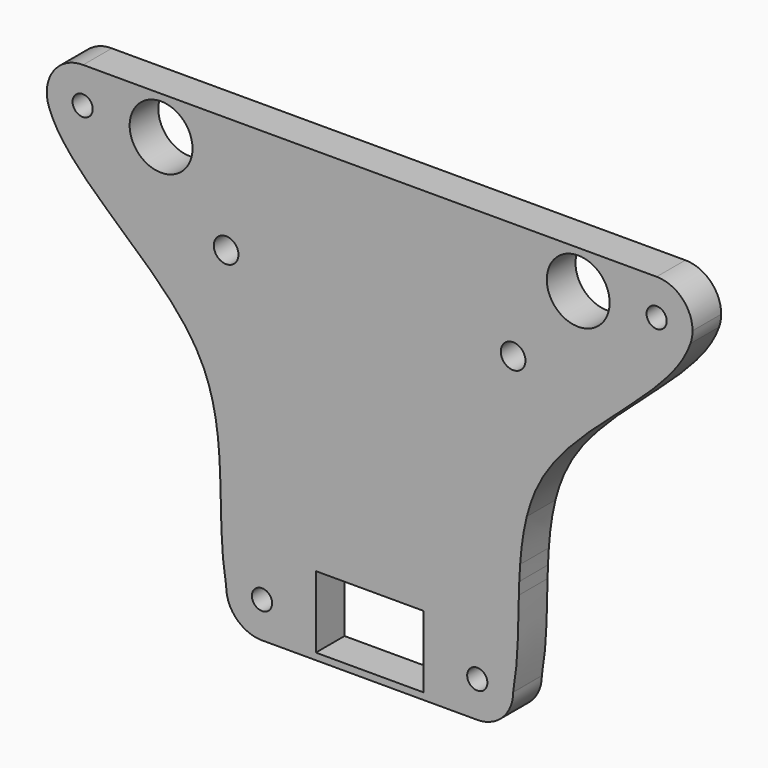
from build123d import *

# Parameters (mm, degrees)
F0_R     = 7.14375
F0_R_2   = 8.73125
F0_R_3   = 22.2504
F0_W     = 76.2
F0_H     = 50.8
F1_DEPTH = 25.4


with BuildPart() as f1:
    # F0 (on Front) → F1 (new body)
    with BuildSketch(Plane.XZ):
        with BuildLine():
            ThreePointArc((-227.1798288962, 117.9559066231), (-198.9530984214, 101.2877007654), (-177.8, 126.3301412811))
            ThreePointArc((-177.8, 126.3301412811), (-185.1223559639, 144.1727528082), (-202.8676209531, 151.7279664669))
            ThreePointArc((-202.8676209531, 151.7279664669), (-223.8140359372, 141.1700038944), (-227.1798288962, 117.9559066231))
        make_face()
        with Locations((-203.2, 126.3301412811)):
            Circle(F0_R, mode=Mode.SUBTRACT)
        with BuildLine():
            ThreePointArc((-202.8676209531, 151.7279664669), (-185.1223559639, 144.1727528082), (-177.8, 126.3301412811))
            ThreePointArc((-177.8, 126.3301412811), (-198.9530984214, 101.2877007654), (-227.1798288962, 117.9559066231))
            add(Edge.make_bspline(
                [(-227.1798288962, 117.9559066231), (-213.6418582626, 78.8128585754), (-134.6303143568, 37.7909136067), (-113.6413747749, -18.1169363843), (-111.2338181852, -27.6559796071)],
                knots=[0, 0, 0, 0, 0.5134678559, 0.6154322526, 0.6154322526, 0.6154322526, 0.6154322526], degree=3))
            Line((-111.2338181852, -27.6559796071), (111.2338181852, -27.6559796071))
            add(Edge.make_bspline(
                [(227.1798288962, 117.9559066231), (213.6418582626, 78.8128585754), (134.6303143568, 37.7909136067), (113.6413747749, -18.1169363843), (111.2338181852, -27.6559796071)],
                knots=[0, 0, 0, 0, 0.5134678559, 0.6154322526, 0.6154322526, 0.6154322526, 0.6154322526], degree=3))
            ThreePointArc((227.1798288962, 117.9559066231), (182.4893469663, 111.6254192192), (203.1998639628, 151.7301412808))
            Line((203.1998639628, 151.7301412808), (-202.8676209531, 151.7279664669))
        make_face()
        with Locations((-101.6, 69.1801412811)):
            Circle(F0_R_2, mode=Mode.SUBTRACT)
        with Locations((-147.6733071194, 124.7280620759)):
            Circle(F0_R_3, mode=Mode.SUBTRACT)
        with Locations((101.6, 69.1801412811)):
            Circle(F0_R_2, mode=Mode.SUBTRACT)
        with Locations((147.6733071194, 124.7280620759)):
            Circle(F0_R_3, mode=Mode.SUBTRACT)
        with BuildLine():
            ThreePointArc((228.6, 126.3301412811), (221.1604641457, 144.2907016196), (203.1998639628, 151.7301412808))
            ThreePointArc((203.1998639628, 151.7301412808), (182.4893469663, 111.6254192192), (227.1798288962, 117.9559066231))
            ThreePointArc((227.1798288962, 117.9559066231), (228.2424405157, 122.0832397026), (228.6, 126.3301412811))
        make_face()
        with Locations((203.2, 126.3301412811)):
            Circle(F0_R, mode=Mode.SUBTRACT)
        with BuildLine():
            Line((111.2338181852, -27.6559796071), (-111.2338181852, -27.6559796071))
            add(Edge.make_bspline(
                [(-111.2338181852, -27.6559796071), (-108.6624430935, -37.8440924207), (-107.3114943085, -48.3473495809), (-106.5439984378, -59.0045117357)],
                knots=[0.6154322526, 0.6154322526, 0.6154322526, 0.6154322526, 0.7243346607, 0.7243346607, 0.7243346607, 0.7243346607], degree=3))
            ThreePointArc((-106.5439984378, -59.0045117357), (-98.7916333235, -57.5943734425), (-94.4499, -64.1698587189))
            ThreePointArc((-94.4499, -64.1698587189), (-98.4312031682, -70.5794341064), (-105.9413914893, -69.8510777735))
            add(Edge.make_bspline(
                [(-105.9413914893, -69.8510777735), (-105.8225617688, -72.7133360171), (-105.7298757075, -75.582653183), (-105.6512856578, -78.4559796071)],
                knots=[0.7611223242, 0.7611223242, 0.7611223242, 0.7611223242, 0.7901378963, 0.7901378963, 0.7901378963, 0.7901378963], degree=3))
            Line((-105.6512856578, -78.4559796071), (105.6512856578, -78.4559796071))
            add(Edge.make_bspline(
                [(105.9413914893, -69.8510777735), (105.8225617688, -72.7133360171), (105.7298757075, -75.582653183), (105.6512856578, -78.4559796071)],
                knots=[0.7611223242, 0.7611223242, 0.7611223242, 0.7611223242, 0.7901378963, 0.7901378963, 0.7901378963, 0.7901378963], degree=3))
            ThreePointArc((105.9413914893, -69.8510777735), (94.4609093557, -63.7732294435), (106.5439984378, -59.0045117357))
            add(Edge.make_bspline(
                [(111.2338181852, -27.6559796071), (108.6624430935, -37.8440924207), (107.3114943085, -48.3473495809), (106.5439984378, -59.0045117357)],
                knots=[0.6154322526, 0.6154322526, 0.6154322526, 0.6154322526, 0.7243346607, 0.7243346607, 0.7243346607, 0.7243346607], degree=3))
        make_face()
        with BuildLine():
            ThreePointArc((-94.4499, -64.1698587189), (-98.7916333235, -57.5943734425), (-106.5439984378, -59.0045117357))
            add(Edge.make_bspline(
                [(-106.5439984378, -59.0045117357), (-106.2847353017, -62.6045431988), (-106.0920508575, -66.2221369929), (-105.9413914893, -69.8510777735)],
                knots=[0.7243346607, 0.7243346607, 0.7243346607, 0.7243346607, 0.7611223242, 0.7611223242, 0.7611223242, 0.7611223242], degree=3))
            ThreePointArc((-105.9413914893, -69.8510777735), (-98.4312031682, -70.5794341064), (-94.4499, -64.1698587189))
        make_face()
        with BuildLine():
            add(Edge.make_bspline(
                [(106.5439984378, -59.0045117357), (106.2847353017, -62.6045431988), (106.0920508575, -66.2221369929), (105.9413914893, -69.8510777735)],
                knots=[0.7243346607, 0.7243346607, 0.7243346607, 0.7243346607, 0.7611223242, 0.7611223242, 0.7611223242, 0.7611223242], degree=3))
            ThreePointArc((106.5439984378, -59.0045117357), (94.4609093557, -63.7732294435), (105.9413914893, -69.8510777735))
        make_face()
        with BuildLine():
            Line((105.6512856578, -78.4559796071), (-105.6512856578, -78.4559796071))
            add(Edge.make_bspline(
                [(-105.6512856578, -78.4559796071), (-105.0828642234, -99.2380039713), (-105.2518408856, -120.2297627942), (-101.5998316324, -140.277376034)],
                knots=[0.7901378963, 0.7901378963, 0.7901378963, 0.7901378963, 1, 1, 1, 1], degree=3))
            ThreePointArc((-101.5998316324, -140.277376034), (-76.1537585809, -114.9699008108), (-50.8, -140.3698587189))
            ThreePointArc((-50.8, -140.3698587189), (-58.1440736415, -158.2344472486), (-75.9294112862, -165.7684173738))
            Line((-75.9294112862, -165.7684173738), (76.1997593484, -165.7698587177))
            ThreePointArc((76.1997593484, -165.7698587177), (58.2069048287, -122.4419886235), (101.5998316324, -140.277376034))
            add(Edge.make_bspline(
                [(105.6512856578, -78.4559796071), (105.0828642234, -99.2380039713), (105.2518408856, -120.2297627942), (101.5998316324, -140.277376034)],
                knots=[0.7901378963, 0.7901378963, 0.7901378963, 0.7901378963, 1, 1, 1, 1], degree=3))
        make_face()
        with Locations((0, -135.6059796071)):
            Rectangle(F0_W, F0_H, mode=Mode.SUBTRACT)
        with BuildLine():
            ThreePointArc((-50.8, -140.3698587189), (-76.1537585809, -114.9699008108), (-101.5998316324, -140.277376034))
            ThreePointArc((-101.5998316324, -140.277376034), (-94.2885883712, -158.2013749399), (-76.4710699897, -165.7684122419))
            Line((-76.4710699897, -165.7684122419), (-75.9294112862, -165.7684173738))
            ThreePointArc((-75.9294112862, -165.7684173738), (-58.1440736415, -158.2344472486), (-50.8, -140.3698587189))
        make_face()
        with Locations((-76.2, -140.3698587189)):
            Circle(F0_R, mode=Mode.SUBTRACT)
        with BuildLine():
            ThreePointArc((101.6, -140.3698587189), (101.5999579081, -140.3236172998), (101.5998316324, -140.277376034))
            ThreePointArc((101.5998316324, -140.277376034), (58.2069048287, -122.4419886235), (76.1997593484, -165.7698587177))
            ThreePointArc((76.1997593484, -165.7698587177), (94.1604271587, -158.330456044), (101.6, -140.3698587189))
        make_face()
        with Locations((76.2, -140.3698587189)):
            Circle(F0_R, mode=Mode.SUBTRACT)
    extrude(amount=F1_DEPTH)


solid = f1.part
